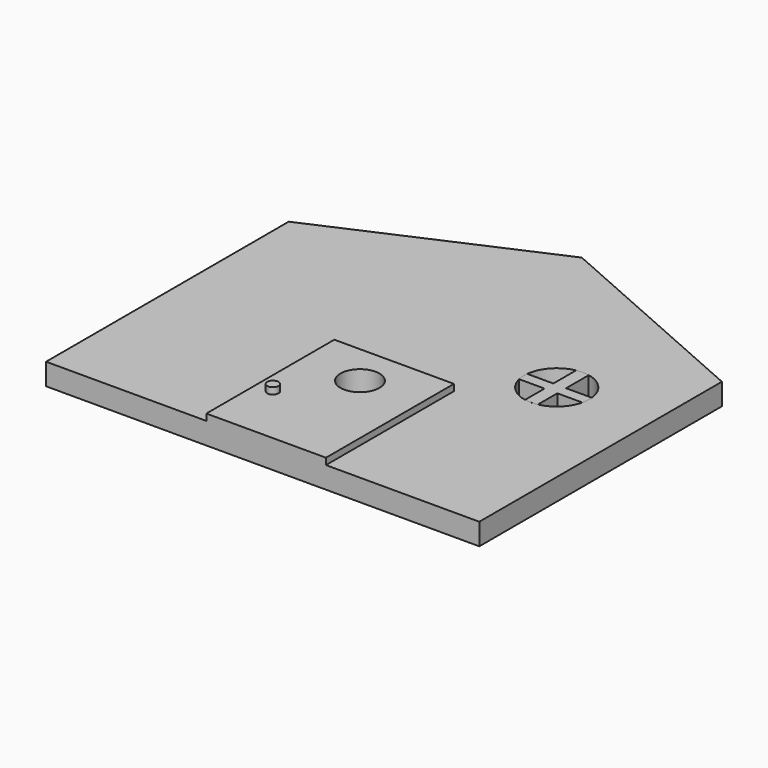
from build123d import *

# Parameters (mm, degrees)
F0_W      = 254
F0_H      = 177.8
F1_DEPTH  = 12.7
F3_D      = 38.1
F4_W      = 70.1176375151
F4_H      = 93.7658244599
F5_DEPTH  = 3.81
F7_D      = 22.86
F9_DEPTH  = 12.7
F8_W      = 7.4963332962
F8_H      = 6.4259641575
F10_DEPTH = 12.7
F11_DEPTH = 12.7
F12_DEPTH = 25.4
F13_DEPTH = 12.7
F14_R     = 3.3045515418
F15_DEPTH = 3.81


with BuildPart() as f1:
    # F0 (on Top) → F1 (new body)
    with BuildSketch(Plane.XY):
        with Locations((-273.1029465795, 124.4398064624)):
            Rectangle(F0_W, F0_H)
        Polygon((-273.1029465795, 269.3603634834), (-400.1029465795, 213.3398064624), (-146.1029465795, 213.3398064624), align=None)
    extrude(amount=F1_DEPTH)

    # F3 (through all)
    with Locations(Plane.XY.offset(12.7)):
        with Locations((-201.6059309244, 161.6795957088)):
            Hole(F3_D / 2)

    # F4 (on face) → F5 (join)
    with BuildSketch(Plane.XY.offset(12.7)):
        with Locations((-271.0681334138, 82.4227186924)):
            Rectangle(F4_W, F4_H)
    extrude(amount=F5_DEPTH)

    # F7 (through all)
    with Locations(Plane.XY.offset(16.51)):
        with Locations((-271.5625464916, 104.8922762275)):
            Hole(F7_D / 2)

    # F14 (on face) → F15 (join)
    with BuildSketch(Plane.XY.offset(16.51)):
        with Locations((-296.1127758026, 71.7939063907)):
            Circle(F14_R)
    extrude(amount=F15_DEPTH)


with BuildPart() as f9:
    # F8 (on face) → F9 (new body)
    with BuildSketch(Plane.XY.offset(12.7)):
        with BuildLine():
            ThreePointArc((-197.7681655949, 180.3390184565), (-201.514545885, 180.7293765153), (-205.2644988911, 180.3749796427))
            Line((-205.2644988911, 180.3749796427), (-205.2644988911, 163.7296213064))
            Line((-205.2644988911, 163.7296213064), (-197.7681655949, 163.7296213064))
            Line((-197.7681655949, 163.7296213064), (-197.7681655949, 180.3390184565))
        make_face()
    extrude(amount=-F9_DEPTH)

    # F8 (on face) → F10 (join)
    with BuildSketch(Plane.XY.offset(12.7)):
        with Locations((-201.516332243, 160.5166392277)):
            Rectangle(F8_W, F8_H)
    extrude(amount=-F10_DEPTH)

    # F8 (on face) → F11 (join)
    with BuildSketch(Plane.XY.offset(12.7)):
        with BuildLine():
            Line((-197.7681655949, 157.3036571489), (-205.2644988911, 157.3036571489))
            Line((-205.2644988911, 157.3036571489), (-205.2644988911, 142.984211775))
            ThreePointArc((-205.2644988911, 142.984211775), (-201.514545885, 142.6298149024), (-197.7681655949, 143.0201729612))
            Line((-197.7681655949, 143.0201729612), (-197.7681655949, 157.3036571489))
        make_face()
    extrude(amount=-F11_DEPTH)

    # F8 (on face) → F12 (join)
    with BuildSketch(Plane.XY.offset(12.7)):
        with BuildLine():
            Line((-182.6665567254, 163.7296213064), (-197.7681655949, 163.7296213064))
            Line((-197.7681655949, 163.7296213064), (-197.7681655949, 157.3036571489))
            Line((-197.7681655949, 157.3036571489), (-183.0653359577, 157.3036571489))
            ThreePointArc((-183.0653359577, 157.3036571489), (-182.6837107307, 159.4768512974), (-182.5559309244, 161.6795957088))
            ThreePointArc((-182.5559309244, 161.6795957088), (-182.5836074794, 162.7060998514), (-182.6665567254, 163.7296213064))
        make_face()
    extrude(amount=-F12_DEPTH)

    # F8 (on face) → F13 (join)
    with BuildSketch(Plane.XY.offset(12.7)):
        with BuildLine():
            Line((-205.2644988911, 157.3036571489), (-205.2644988911, 163.7296213064))
            Line((-205.2644988911, 163.7296213064), (-220.5453051234, 163.7296213064))
            ThreePointArc((-220.5453051234, 163.7296213064), (-220.6193544984, 160.4996702891), (-220.1465258911, 157.3036571489))
            Line((-220.1465258911, 157.3036571489), (-205.2644988911, 157.3036571489))
        make_face()
    extrude(amount=-F13_DEPTH)


solid = Compound([f1.part, f9.part])
